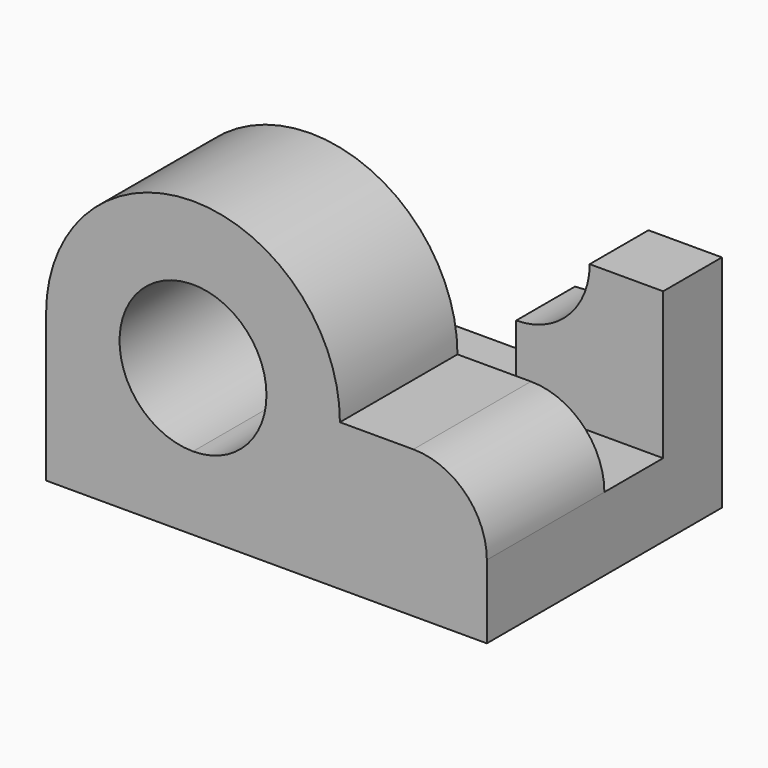
from build123d import *

# Parameters (mm, degrees)
F0_W     = 60
F0_H     = 40
F1_DEPTH = 10
F3_DEPTH = 20
F5_DEPTH = 25
F7_DEPTH = 10
F8_R     = 9.99999


# Not quite as in the source:
# - a fillet or chamfer is up to 0.001 mm smaller than in the source, because OpenCascade refuses the exact size


with BuildPart() as f1:
    # F0 (on Top) → F1 (new body)
    with BuildSketch(Plane.XY):
        with Locations((30, 20)):
            Rectangle(F0_W, F0_H)
    extrude(amount=F1_DEPTH)

    # F2 (on Front) → F3 (join)
    with BuildSketch(Plane.XZ):
        with BuildLine():
            Line((50, 20), (40, 20))
            ThreePointArc((40, 20), (20, 40), (0, 20))
            Line((0, 20), (0, 10))
            Line((0, 10), (60, 10))
            ThreePointArc((60, 10), (57.0710678119, 17.0710678119), (50, 20))
        make_face()
    extrude(amount=-F3_DEPTH)

    # F4 (on face) → F5 (cut)
    with BuildSketch(Plane.XZ):
        with BuildLine():
            ThreePointArc((30, 20), (12.928932207, 27.0710678307), (19.9999999466, 10))
            ThreePointArc((19.9999999466, 10), (27.071067793, 12.9289321693), (30, 20))
        make_face()
    extrude(amount=-F5_DEPTH, mode=Mode.SUBTRACT)

    # F6 (on face) → F7 (join)
    with BuildSketch(Plane(origin=(0, 40, 0), x_dir=(-1, 0, 0), z_dir=(0, 1, 0))):
        Polygon((-60, 30), (-60, 10), (-40, 10), (-40, 20), (-50, 20), (-50, 30), align=None)
    extrude(amount=-F7_DEPTH)

    # F8 (radius 10 in the source; OpenCascade refuses exactly that, so slightly less here)
    f8_edges = [f1.edges().sort_by_distance(p)[0] for p in [
        (50, 35, 20),
    ]]
    fillet(f8_edges, radius=F8_R)


solid = f1.part
